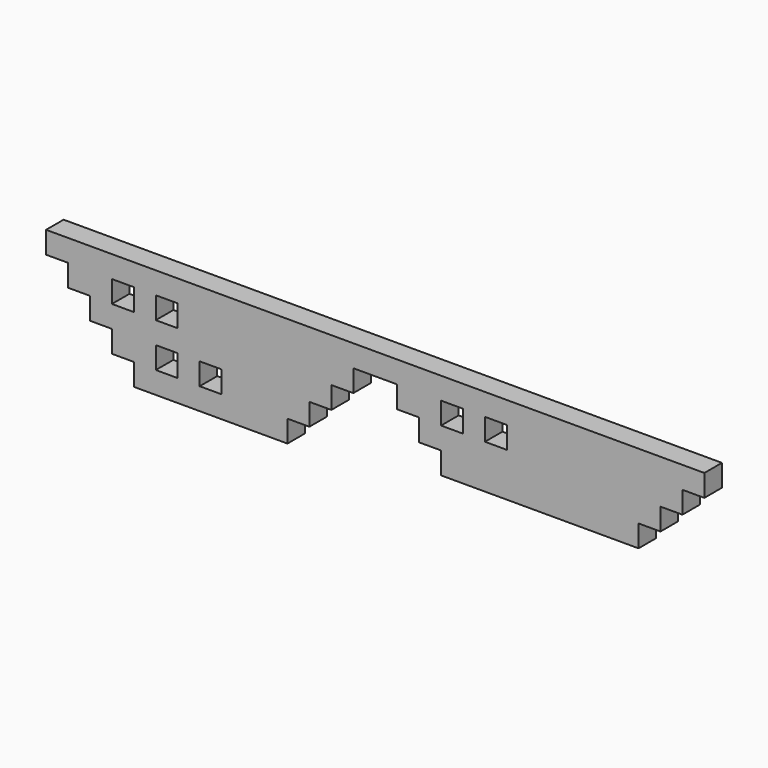
from build123d import *

# Parameters (mm, degrees)
F0_W     = 5.08
F0_H     = 5.08
F1_DEPTH = 5.08


# Not quite as in the source:
# - a feature names something its author has since deleted; it is built from what else it names


with BuildPart() as f1:
    # F0 (on Front) → F1 (new body)
    with BuildSketch(Plane.XZ):
        Polygon((0, 5.08), (0, 10.16), (-76.2, 10.16), (-76.2, 5.08), (-71.12, 5.08), (-71.12, 0), (-66.04, 0), (-66.04, -5.08), (-60.96, -5.08), (-60.96, -10.16), (-55.88, -10.16), (-55.88, -15.24), (-20.32, -15.24), (-20.32, -10.16), (-15.24, -10.16), (-15.24, -5.08), (-10.16, -5.08), (-10.16, 0), (-5.08, 0), (-5.08, 5.08), align=None)
        with Locations((-48.26, -7.62)):
            Rectangle(F0_W, F0_H, mode=Mode.SUBTRACT)
        with Locations((-38.1, -7.62)):
            Rectangle(F0_W, F0_H, mode=Mode.SUBTRACT)
        with Locations((-58.42, 2.54)):
            Rectangle(F0_W, F0_H, mode=Mode.SUBTRACT)
        with Locations((-48.26, 2.54)):
            Rectangle(F0_W, F0_H, mode=Mode.SUBTRACT)
        Polygon((76.2, 10.16), (0, 10.16), (0, 5.08), (5.08, 5.08), (5.08, 0), (10.16, 0), (10.16, -5.08), (15.24, -5.08), (15.24, -10.16), (20.32, -10.16), (55.88, -10.16), (60.96, -10.16), (60.96, -5.08), (66.04, -5.08), (66.04, 0), (71.12, 0), (71.12, 5.08), (76.2, 5.08), align=None)
        with Locations((17.78, 2.54)):
            Rectangle(F0_W, F0_H, mode=Mode.SUBTRACT)
        with Locations((27.94, 2.54)):
            Rectangle(F0_W, F0_H, mode=Mode.SUBTRACT)
    extrude(amount=-F1_DEPTH)


solid = f1.part
